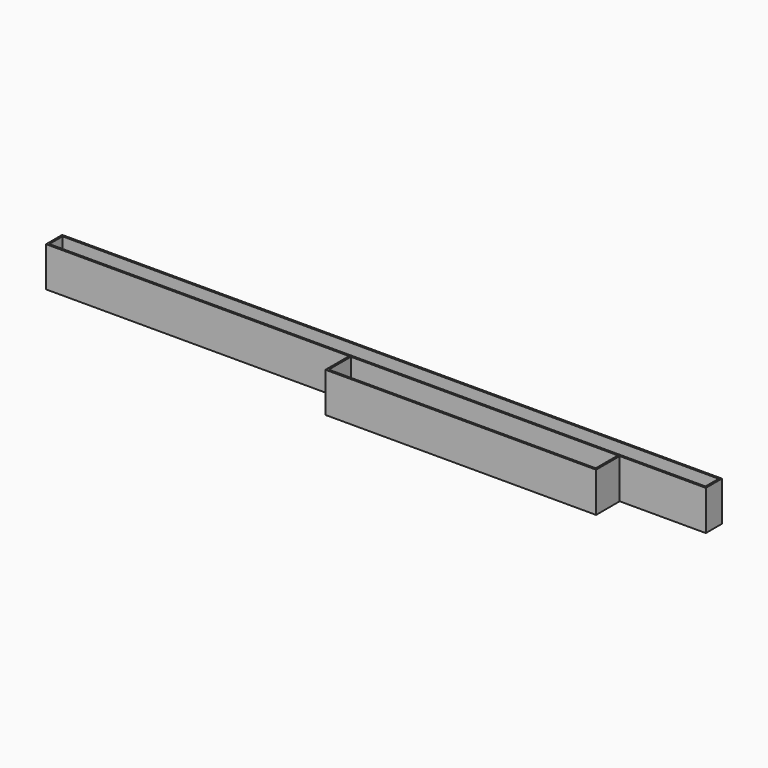
from build123d import *

# Parameters (mm, degrees)
F2_W     = 0.8
F2_H     = 7.4
F2_W_2   = 121
F2_H_2   = 13.2
F3_DEPTH = 17.8
F4_T     = -0.8


# Not quite as in the source:
# - a shell that OpenCascade refuses in one call is made with other operations: the cavity is built on its own and cut out


with BuildPart() as f3:
    # F2 (on Top) → F3 (new body)
    with BuildSketch(Plane.XY):
        Polygon((-135.5, 9), (-135.5, 8.2), (-134.7, 8.2), (158.7, 8.2), (159.5, 8.2), (159.5, 9), align=None)
        with Locations((159.1, 4.5)):
            Rectangle(F2_W, F2_H)
        with Locations((-135.1, 4.5)):
            Rectangle(F2_W, F2_H)
        with Locations((60.5, -6.6)):
            Rectangle(F2_W_2, F2_H_2)
        Polygon((-135.5, 0), (0, 0), (121, 0), (159.5, 0), (159.5, 0.8), (158.7, 0.8), (-134.7, 0.8), (-135.5, 0.8), align=None)
    extrude(amount=F3_DEPTH)

    # F4: a shell. OpenCascade refuses it in one call, so the cavity is built on its own and cut out:
    # the body offset inwards by the wall thickness, plus a prism from it out through each open face.
    f4_core = offset(f3.part, amount=F4_T, kind=Kind.INTERSECTION, mode=Mode.PRIVATE)
    f4_exits = [f4_core.faces().sort_by_distance(p)[0] for p in [
        (60.5, -6.2, 17),
    ]]
    add(f4_core, mode=Mode.SUBTRACT)
    extrude(f4_exits, amount=-F4_T, mode=Mode.SUBTRACT)


solid = f3.part
